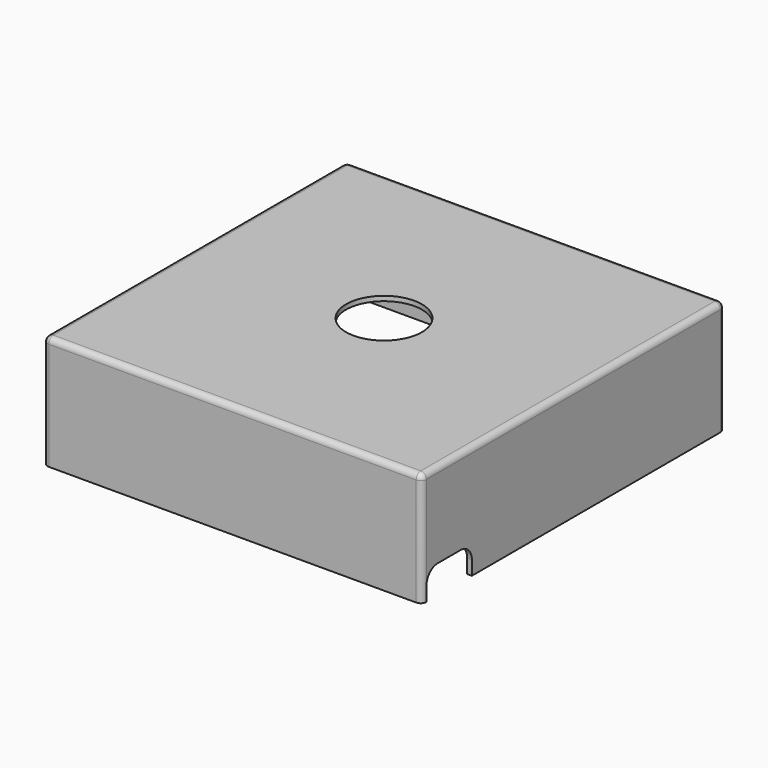
from build123d import *

# Parameters (mm, degrees)
F0_W          = 200
F0_H          = 200
F0_R          = 20
F1_DEPTH      = 60
F2_R          = 3
F3_T          = -2.5
F4_DEPTH      = 60
F6_DEPTH      = 25
F8_DEPTH      = 25
F9_DEPTH      = 2
F9_DEPTH_BACK = 4
F10_T1_DEPTH  = 7.5
F10_T4_ANGLE  = 180
F10_T6_ANGLE  = 180


# Not quite as in the source:
# - a fillet or chamfer that OpenCascade refuses, or shapes differently, is made with other operations: its cross-section is extruded or revolved along the edge and cut away or added


with BuildPart() as f1:
    # F0 (on Top) → F1 (new body)
    with BuildSketch(Plane.XY):
        with Locations((100, -100)):
            Rectangle(F0_W, F0_H)
        with Locations((100, -100)):
            Circle(F0_R, mode=Mode.SUBTRACT)
        with Locations((100, -100)):
            Circle(F0_R)
    extrude(amount=F1_DEPTH)

    # F2
    f2_edges = [f1.edges().sort_by_distance(p)[0] for p in [
        (100, 0, 60),
        (200, -100, 60),
        (100, -200, 60),
        (0, -100, 60),
        (0, 0, 30),
        (0, -200, 30),
        (200, -200, 30),
        (200, 0, 30),
    ]]
    fillet(f2_edges, radius=F2_R)

    # F3
    f3_openings = [f1.faces().sort_by_distance(p)[0] for p in [
        (100, -100, 0),
    ]]
    offset(amount=F3_T, openings=f3_openings)

    # F0 (on Top) → F4 (cut, through all)
    with BuildSketch(Plane.XY):
        with Locations((100, -100)):
            Circle(F0_R)
    extrude(amount=F4_DEPTH, mode=Mode.SUBTRACT)

    # F5 (on face) → F6 (cut)
    with BuildSketch(Plane.YZ.offset(200)):
        with BuildLine():
            Line((-197, 7.5), (-197, 0))
            Line((-197, 0), (-167, 0))
            Line((-167, 0), (-167, 7.5))
            ThreePointArc((-167, 7.5), (-169.1966991411, 12.8033008589), (-174.5, 15))
            Line((-174.5, 15), (-189.5, 15))
            ThreePointArc((-189.5, 15), (-194.8033008589, 12.8033008589), (-197, 7.5))
        make_face()
    extrude(amount=-F6_DEPTH, mode=Mode.SUBTRACT)

    # F7 (on face) → F8 (cut)
    with BuildSketch(Plane(origin=(0, 0, 0), x_dir=(-1, 0, 0), z_dir=(0, 1, 0))):
        with BuildLine():
            Line((-92.5, 0), (-92.5, 7.5))
            ThreePointArc((-92.5, 7.5), (-100, 15), (-107.5, 7.5))
            Line((-107.5, 7.5), (-107.5, 0))
            Line((-107.5, 0), (-92.5, 0))
        make_face()
    extrude(amount=-F8_DEPTH, mode=Mode.SUBTRACT)

    # F7 (on face) → F9 (join, two sides)
    with BuildSketch(Plane(origin=(0, 0, 0), x_dir=(-1, 0, 0), z_dir=(0, 1, 0))) as f9_sk:
        with BuildLine():
            ThreePointArc((-107.5, 7.5), (-100, 15), (-92.5, 7.5))
            Line((-92.5, 7.5), (-92.5, 0))
            Line((-92.5, 0), (-87.5, 0))
            Line((-87.5, 0), (-87.5, 7.5))
            ThreePointArc((-87.5, 7.5), (-100, 20), (-112.5, 7.5))
            Line((-112.5, 7.5), (-112.5, 0))
            Line((-112.5, 0), (-107.5, 0))
            Line((-107.5, 0), (-107.5, 7.5))
        make_face()
    extrude(amount=F9_DEPTH)
    extrude(f9_sk.sketch, amount=-F9_DEPTH_BACK)

    # F10: fillet of radius 5 on 2 edges, made by hand

    # F10_s2 → F10_t1 (join)
    with BuildSketch(Plane.XY):
        with BuildLine():
            ThreePointArc((116.0707142143, -2.5), (114.1342225412, -2.8902277714), (112.5, -4))
            Line((112.5, -4), (112.5, -2.5))
            Line((112.5, -2.5), (116.0707142143, -2.5))
        make_face()
        with BuildLine():
            ThreePointArc((83.9292857857, -2.5), (85.8657774588, -2.8902277714), (87.5, -4))
            Line((87.5, -4), (87.5, -2.5))
            Line((87.5, -2.5), (83.9292857857, -2.5))
        make_face()
        with BuildLine():
            ThreePointArc((116.5, 0), (114.2639320225, 0.527864045), (112.5, 2))
            Line((112.5, 2), (112.5, 0))
            Line((112.5, 0), (116.5, 0))
        make_face()
        with BuildLine():
            ThreePointArc((83.5, 0), (85.7360679775, 0.527864045), (87.5, 2))
            Line((87.5, 2), (87.5, 0))
            Line((87.5, 0), (83.5, 0))
        make_face()
    extrude(amount=F10_T1_DEPTH)

    # F10_s3 → F10_t4 (revolve)
    with BuildSketch(Plane.XY.offset(7.5)):
        with BuildLine():
            ThreePointArc((116.5, 0), (114.2639320225, 0.527864045), (112.5, 2))
            Line((112.5, 2), (112.5, 0))
            Line((112.5, 0), (116.5, 0))
        make_face()
    revolve(axis=Axis((100, 0, 7.5), (0, -1, 0)), revolution_arc=F10_T4_ANGLE)

    # F10_s5 → F10_t6 (revolve)
    with BuildSketch(Plane.XY.offset(7.5)):
        with BuildLine():
            ThreePointArc((116.0707142143, -2.5), (114.1342225412, -2.8902277714), (112.5, -4))
            Line((112.5, -4), (112.5, -2.5))
            Line((112.5, -2.5), (116.0707142143, -2.5))
        make_face()
    revolve(axis=Axis((100, -2.5, 7.5), (0, -1, 0)), revolution_arc=F10_T6_ANGLE)


solid = f1.part
